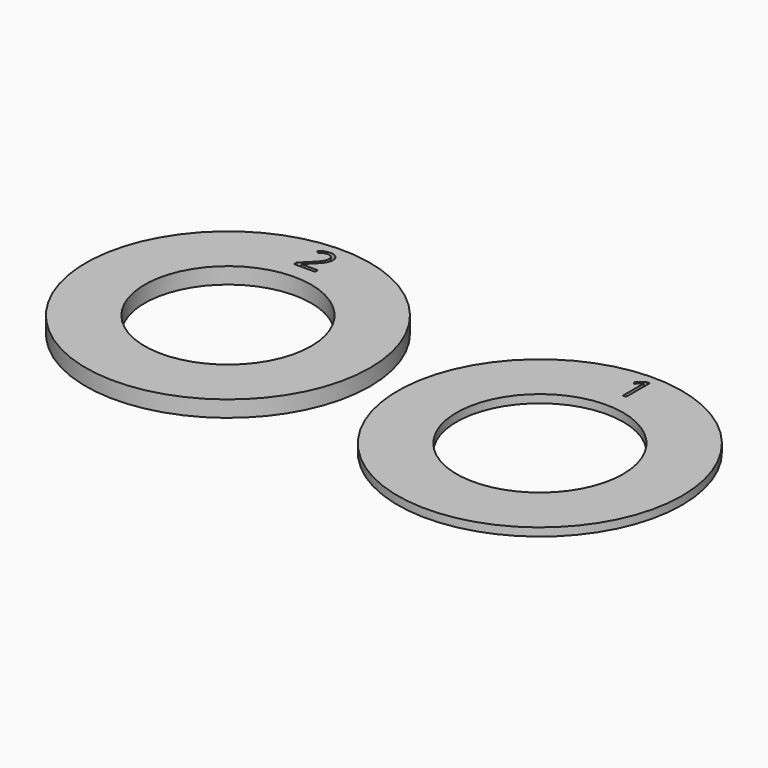
from build123d import *

# Parameters (mm, degrees)
F0_R         = 17.5
F0_R_2       = 10.25
F1_DEPTH     = 2
F2_TEXT_SIZE = 5.5326045387
F3_DEPTH     = 2
F4_R         = 17.5
F4_R_2       = 10.25
F5_DEPTH     = 1
F6_TEXT_SIZE = 5.0938274297
F7_DEPTH     = 1


# Not quite as in the source:
# - Text() gives the source's letters only with a copy of the font that has no kerning and outlines rounded to 1/6400 em; it was checked with that copy


with BuildPart() as f1:
    # F0 (on Top) → F1 (new body)
    with BuildSketch(Plane.XY):
        with Locations((-32.9609513283, 29.3432921171)):
            Circle(F0_R)
        with Locations((-32.9609513283, 29.3432921171)):
            Circle(F0_R_2, mode=Mode.SUBTRACT)
    extrude(amount=F1_DEPTH)

    # F2 (on face) → F3 (cut)
    with BuildSketch(Plane.XY.offset(2)):
        with Locations((-34.9526852369, 41.6522286832)):
            Text('2', F2_TEXT_SIZE, font='Open Sans', text_align=(TextAlign.LEFT, TextAlign.BOTTOM))
    extrude(amount=-F3_DEPTH, mode=Mode.SUBTRACT)


with BuildPart() as f5:
    # F4 (on Top) → F5 (new body)
    with BuildSketch(Plane.XY):
        with Locations((5.8893924579, 28.7736225873)):
            Circle(F4_R)
        with Locations((5.8893924579, 28.7736225873)):
            Circle(F4_R_2, mode=Mode.SUBTRACT)
    extrude(amount=F5_DEPTH)

    # F6 (on face) → F7 (cut)
    with BuildSketch(Plane.XY.offset(1)):
        with Locations((4.5358522329, 41.5126718581)):
            Text('1', F6_TEXT_SIZE, font='Open Sans', text_align=(TextAlign.LEFT, TextAlign.BOTTOM))
    extrude(amount=-F7_DEPTH, mode=Mode.SUBTRACT)


solid = Compound([f1.part, f5.part])
